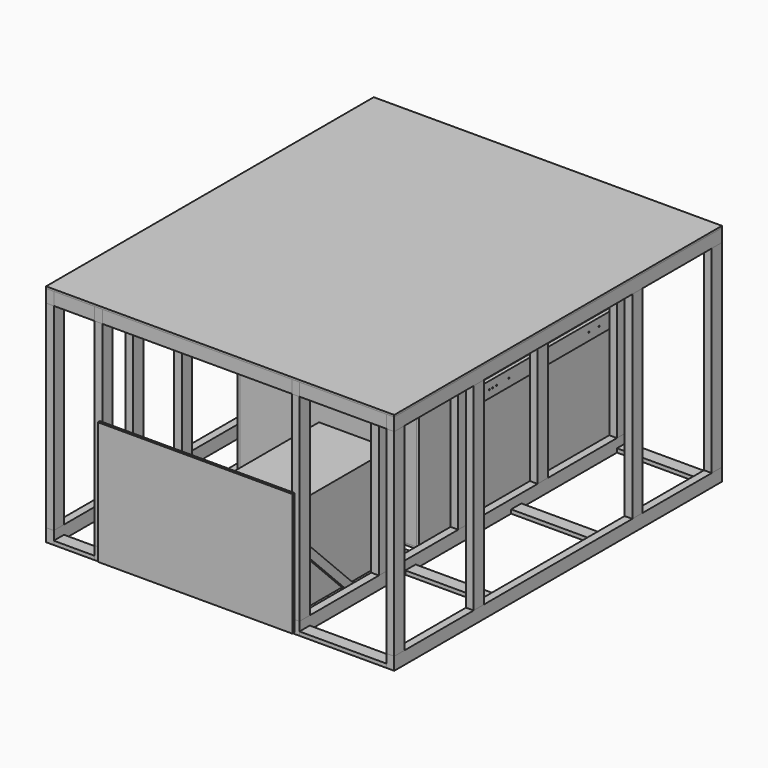
from build123d import *

# Parameters (mm, degrees)
F1_W            = 1727.2
F1_H            = 2032
F2_DEPTH        = 9.525
F3_W            = 38.1
F3_H            = 63.5
F4_DEPTH        = 2032
F5_W            = 38.1
F5_H            = 63.5
F6_DEPTH        = 981.075
F7_W            = 63.5
F7_H            = 19.05
F8_DEPTH        = 203.2
F7_W_2          = 38.1
F7_H_2          = 63.5
F7_W_3          = 19.05
F8_COPIES_COUNT = 3
F8_COPIES_PITCH = 656.166667
F9_W            = 63.5
F9_H            = 19.05
F10_DEPTH       = 431.8
F9_W_2          = 38.1
F9_H_2          = 63.5
F9_W_3          = 19.05
F11_W           = 63.5
F11_H           = 19.05
F12_DEPTH       = 939.8
F11_W_2         = 38.1
F11_H_2         = 63.5
F11_W_3         = 19.05
F13_W           = 19.05
F13_H           = 76.2
F14_DEPTH       = 914.4
F15_R           = 3.302
F16_DEPTH       = 19.05
F16_DEPTH_BACK  = 920.75
F17_W           = 901.7
F17_H           = 9.525
F18_DEPTH       = 1219.2
F19_W           = 12.7
F19_H           = 1219.2
F20_DEPTH       = 609.6
F19_W_2         = 875.792
F19_H_2         = 12.7
F21_W           = 762
F21_H           = 266.7
F22_DEPTH       = 1219.2
F24_DEPTH       = 914.4
F25_W           = 927.1
F25_H           = 9.525
F26_DEPTH       = 762
F27_W           = 965.2
F27_H           = 609.6
F28_DEPTH       = 12.7
F29_W           = 355.6
F29_H           = 635
F30_DEPTH       = 482.6
F32_DEPTH       = 19.05


# Not quite as in the source:
# - a pattern or mirror of a feature is missing from the dataset's text; its kind, count and spacing are read off the source's solid


with BuildPart() as f2:
    # F1 (on offset) → F2 (new body)
    with BuildSketch(Plane.XY.offset(1117.6)):
        Rectangle(F1_W, F1_H)
    extrude(amount=-F2_DEPTH)


with BuildPart() as f4:
    # F3 (on face) → F4 (new body, through all)
    with BuildSketch(Plane(origin=(0, 1016, 0), x_dir=(-1, 0, 0), z_dir=(0, 1, 0))):
        with Locations((-844.55, 1076.325)):
            Rectangle(F3_W, F3_H)
    extrude(amount=-F4_DEPTH)


with BuildPart() as f4b:
    # F3 (on face) → F4, piece 2 (new body, through all)
    with BuildSketch(Plane(origin=(0, 1016, 0), x_dir=(-1, 0, 0), z_dir=(0, 1, 0))):
        with Locations((844.55, 1076.325)):
            Rectangle(F3_W, F3_H)
    extrude(amount=-F4_DEPTH)


with BuildPart() as f4c:
    # F3 (on face) → F4, piece 3 (new body, through all)
    with BuildSketch(Plane(origin=(0, 1016, 0), x_dir=(-1, 0, 0), z_dir=(0, 1, 0))):
        with Locations((-844.55, 31.75)):
            Rectangle(F3_W, F3_H)
    extrude(amount=-F4_DEPTH)


with BuildPart() as f4d:
    # F3 (on face) → F4, piece 4 (new body, through all)
    with BuildSketch(Plane(origin=(0, 1016, 0), x_dir=(-1, 0, 0), z_dir=(0, 1, 0))):
        with Locations((844.55, 31.75)):
            Rectangle(F3_W, F3_H)
    extrude(amount=-F4_DEPTH)


with BuildPart() as f4e:
    # F3 (on face) → F4, piece 5 (new body, through all)
    with BuildSketch(Plane(origin=(0, 1016, 0), x_dir=(-1, 0, 0), z_dir=(0, 1, 0))):
        with Locations((-374.65, 1076.325)):
            Rectangle(F3_W, F3_H)
    extrude(amount=-F4_DEPTH)


with BuildPart() as f4f:
    # F3 (on face) → F4, piece 6 (new body, through all)
    with BuildSketch(Plane(origin=(0, 1016, 0), x_dir=(-1, 0, 0), z_dir=(0, 1, 0))):
        with Locations((603.25, 1076.325)):
            Rectangle(F3_W, F3_H)
    extrude(amount=-F4_DEPTH)


with BuildPart() as f4g:
    # F3 (on face) → F4, piece 7 (new body, through all)
    with BuildSketch(Plane(origin=(0, 1016, 0), x_dir=(-1, 0, 0), z_dir=(0, 1, 0))):
        with Locations((-374.65, 31.75)):
            Rectangle(F3_W, F3_H)
    extrude(amount=-F4_DEPTH)


with BuildPart() as f4h:
    # F3 (on face) → F4, piece 8 (new body, through all)
    with BuildSketch(Plane(origin=(0, 1016, 0), x_dir=(-1, 0, 0), z_dir=(0, 1, 0))):
        with Locations((603.25, 31.75)):
            Rectangle(F3_W, F3_H)
    extrude(amount=-F4_DEPTH)


with BuildPart() as f6:
    # F5 (on face) → F6 (new body, through all)
    with BuildSketch(Plane.XY.offset(63.5)):
        with Locations((844.55, 984.25)):
            Rectangle(F5_W, F5_H)
    extrude(amount=F6_DEPTH)


with BuildPart() as f6b:
    # F5 (on face) → F6, piece 2 (new body, through all)
    with BuildSketch(Plane.XY.offset(63.5)):
        with Locations((844.55, 492.125)):
            Rectangle(F5_W, F5_H)
    extrude(amount=F6_DEPTH)


with BuildPart() as f6c:
    # F5 (on face) → F6, piece 3 (new body, through all)
    with BuildSketch(Plane.XY.offset(63.5)):
        with Locations((844.55, -492.125)):
            Rectangle(F5_W, F5_H)
    extrude(amount=F6_DEPTH)


with BuildPart() as f6d:
    # F5 (on face) → F6, piece 4 (new body, through all)
    with BuildSketch(Plane.XY.offset(63.5)):
        with Locations((844.55, -984.25)):
            Rectangle(F5_W, F5_H)
    extrude(amount=F6_DEPTH)


with BuildPart() as f6e:
    # F5 (on face) → F6, piece 5 (new body, through all)
    with BuildSketch(Plane.XY.offset(63.5)):
        with Locations((374.65, 984.25)):
            Rectangle(F5_W, F5_H)
    extrude(amount=F6_DEPTH)


with BuildPart() as f6f:
    # F5 (on face) → F6, piece 6 (new body, through all)
    with BuildSketch(Plane.XY.offset(63.5)):
        with Locations((374.65, 492.125)):
            Rectangle(F5_W, F5_H)
    extrude(amount=F6_DEPTH)


with BuildPart() as f6g:
    # F5 (on face) → F6, piece 7 (new body, through all)
    with BuildSketch(Plane.XY.offset(63.5)):
        with Locations((374.65, 0)):
            Rectangle(F5_W, F5_H)
    extrude(amount=F6_DEPTH)


with BuildPart() as f6h:
    # F5 (on face) → F6, piece 8 (new body, through all)
    with BuildSketch(Plane.XY.offset(63.5)):
        with Locations((374.65, -492.125)):
            Rectangle(F5_W, F5_H)
    extrude(amount=F6_DEPTH)


with BuildPart() as f6i:
    # F5 (on face) → F6, piece 9 (new body, through all)
    with BuildSketch(Plane.XY.offset(63.5)):
        with Locations((374.65, -984.25)):
            Rectangle(F5_W, F5_H)
    extrude(amount=F6_DEPTH)


with BuildPart() as f6j:
    # F5 (on face) → F6, piece 10 (new body, through all)
    with BuildSketch(Plane.XY.offset(63.5)):
        with Locations((-603.25, 984.25)):
            Rectangle(F5_W, F5_H)
    extrude(amount=F6_DEPTH)


with BuildPart() as f6k:
    # F5 (on face) → F6, piece 11 (new body, through all)
    with BuildSketch(Plane.XY.offset(63.5)):
        with Locations((-603.25, 492.125)):
            Rectangle(F5_W, F5_H)
    extrude(amount=F6_DEPTH)


with BuildPart() as f6l:
    # F5 (on face) → F6, piece 12 (new body, through all)
    with BuildSketch(Plane.XY.offset(63.5)):
        with Locations((-603.25, 0)):
            Rectangle(F5_W, F5_H)
    extrude(amount=F6_DEPTH)


with BuildPart() as f6m:
    # F5 (on face) → F6, piece 13 (new body, through all)
    with BuildSketch(Plane.XY.offset(63.5)):
        with Locations((-603.25, -492.125)):
            Rectangle(F5_W, F5_H)
    extrude(amount=F6_DEPTH)


with BuildPart() as f6n:
    # F5 (on face) → F6, piece 14 (new body, through all)
    with BuildSketch(Plane.XY.offset(63.5)):
        with Locations((-603.25, -984.25)):
            Rectangle(F5_W, F5_H)
    extrude(amount=F6_DEPTH)


with BuildPart() as f6o:
    # F5 (on face) → F6, piece 15 (new body, through all)
    with BuildSketch(Plane.XY.offset(63.5)):
        with Locations((-844.55, 984.25)):
            Rectangle(F5_W, F5_H)
    extrude(amount=F6_DEPTH)


with BuildPart() as f6p:
    # F5 (on face) → F6, piece 16 (new body, through all)
    with BuildSketch(Plane.XY.offset(63.5)):
        with Locations((-844.55, 492.125)):
            Rectangle(F5_W, F5_H)
    extrude(amount=F6_DEPTH)


with BuildPart() as f6q:
    # F5 (on face) → F6, piece 17 (new body, through all)
    with BuildSketch(Plane.XY.offset(63.5)):
        with Locations((-844.55, -492.125)):
            Rectangle(F5_W, F5_H)
    extrude(amount=F6_DEPTH)


with BuildPart() as f6r:
    # F5 (on face) → F6, piece 18 (new body, through all)
    with BuildSketch(Plane.XY.offset(63.5)):
        with Locations((-844.55, -984.25)):
            Rectangle(F5_W, F5_H)
    extrude(amount=F6_DEPTH)


with BuildPart() as f8:
    # F7 (on face) → F8 (new body, through all)
    with BuildSketch(Plane(origin=(-622.3, 0, 0), x_dir=(0, -1, 0), z_dir=(-1, 0, 0))):
        with Locations((-328.0833333333, 9.525)):
            Rectangle(F7_W, F7_H)
    extrude(amount=F8_DEPTH)


with BuildPart() as f8b:
    # F7 (on face) → F8, piece 2 (new body, through all)
    with BuildSketch(Plane(origin=(-622.3, 0, 0), x_dir=(0, -1, 0), z_dir=(-1, 0, 0))):
        with Locations((-984.25, 9.525)):
            Rectangle(F7_W, F7_H)
    extrude(amount=F8_DEPTH)


with BuildPart() as f8c:
    # F7 (on face) → F8, piece 3 (new body, through all)
    with BuildSketch(Plane(origin=(-622.3, 0, 0), x_dir=(0, -1, 0), z_dir=(-1, 0, 0))):
        with Locations((996.95, 1076.325)):
            Rectangle(F7_W_2, F7_H_2)
    extrude(amount=F8_DEPTH)


with BuildPart() as f8d:
    # F7 (on face) → F8, piece 4 (new body, through all)
    with BuildSketch(Plane(origin=(-622.3, 0, 0), x_dir=(0, -1, 0), z_dir=(-1, 0, 0))):
        with Locations((661.4583333333, 1076.325)):
            Rectangle(F7_W_3, F7_H_2)
    extrude(amount=F8_DEPTH)


with BuildPart() as f8e:
    # F7 (on face) → F8, piece 5 (new body, through all)
    with BuildSketch(Plane(origin=(-622.3, 0, 0), x_dir=(0, -1, 0), z_dir=(-1, 0, 0))):
        with Locations((335.4916666667, 1076.325)):
            Rectangle(F7_W_3, F7_H_2)
    extrude(amount=F8_DEPTH)


with BuildPart() as f8f:
    # F7 (on face) → F8, piece 6 (new body, through all)
    with BuildSketch(Plane(origin=(-622.3, 0, 0), x_dir=(0, -1, 0), z_dir=(-1, 0, 0))):
        with Locations((0, 1076.325)):
            Rectangle(F7_W_2, F7_H_2)
    extrude(amount=F8_DEPTH)


with BuildPart() as f8g:
    # F7 (on face) → F8, piece 7 (new body, through all)
    with BuildSketch(Plane(origin=(-622.3, 0, 0), x_dir=(0, -1, 0), z_dir=(-1, 0, 0))):
        with Locations((-335.4916666667, 1076.325)):
            Rectangle(F7_W_3, F7_H_2)
    extrude(amount=F8_DEPTH)


with BuildPart() as f8h:
    # F7 (on face) → F8, piece 8 (new body, through all)
    with BuildSketch(Plane(origin=(-622.3, 0, 0), x_dir=(0, -1, 0), z_dir=(-1, 0, 0))):
        with Locations((-661.4583333333, 1076.325)):
            Rectangle(F7_W_3, F7_H_2)
    extrude(amount=F8_DEPTH)


with BuildPart() as f8i:
    # F7 (on face) → F8, piece 9 (new body, through all)
    with BuildSketch(Plane(origin=(-622.3, 0, 0), x_dir=(0, -1, 0), z_dir=(-1, 0, 0))):
        with Locations((-996.95, 1076.325)):
            Rectangle(F7_W_2, F7_H_2)
    extrude(amount=F8_DEPTH)


with BuildPart() as f8_copies_1:
    # F8_copies: instance of F8
    add(f8.part.moved(Location(Vector(0, -1, 0) * (1 * F8_COPIES_PITCH))))


with BuildPart() as f8_copies_2:
    # F8_copies: instance of F8
    add(f8.part.moved(Location(Vector(0, -1, 0) * (2 * F8_COPIES_PITCH))))


with BuildPart() as f10:
    # F9 (on face) → F10 (new body, through all)
    with BuildSketch(Plane.YZ.offset(393.7)):
        with Locations((-984.25, 9.525)):
            Rectangle(F9_W, F9_H)
    extrude(amount=F10_DEPTH)


with BuildPart() as f10b:
    # F9 (on face) → F10, piece 2 (new body, through all)
    with BuildSketch(Plane.YZ.offset(393.7)):
        with Locations((984.25, 9.525)):
            Rectangle(F9_W, F9_H)
    extrude(amount=F10_DEPTH)


with BuildPart() as f10c:
    # F9 (on face) → F10, piece 3 (new body, through all)
    with BuildSketch(Plane.YZ.offset(393.7)):
        with Locations((328.0833333333, 9.525)):
            Rectangle(F9_W, F9_H)
    extrude(amount=F10_DEPTH)


with BuildPart() as f10d:
    # F9 (on face) → F10, piece 4 (new body, through all)
    with BuildSketch(Plane.YZ.offset(393.7)):
        with Locations((-328.0833333333, 9.525)):
            Rectangle(F9_W, F9_H)
    extrude(amount=F10_DEPTH)


with BuildPart() as f10e:
    # F9 (on face) → F10, piece 5 (new body, through all)
    with BuildSketch(Plane.YZ.offset(393.7)):
        with Locations((996.95, 1076.325)):
            Rectangle(F9_W_2, F9_H_2)
    extrude(amount=F10_DEPTH)


with BuildPart() as f10f:
    # F9 (on face) → F10, piece 6 (new body, through all)
    with BuildSketch(Plane.YZ.offset(393.7)):
        with Locations((661.4583333333, 1076.325)):
            Rectangle(F9_W_3, F9_H_2)
    extrude(amount=F10_DEPTH)


with BuildPart() as f10g:
    # F9 (on face) → F10, piece 7 (new body, through all)
    with BuildSketch(Plane.YZ.offset(393.7)):
        with Locations((335.4916666667, 1076.325)):
            Rectangle(F9_W_3, F9_H_2)
    extrude(amount=F10_DEPTH)


with BuildPart() as f10h:
    # F9 (on face) → F10, piece 8 (new body, through all)
    with BuildSketch(Plane.YZ.offset(393.7)):
        with Locations((0, 1076.325)):
            Rectangle(F9_W_2, F9_H_2)
    extrude(amount=F10_DEPTH)


with BuildPart() as f10i:
    # F9 (on face) → F10, piece 9 (new body, through all)
    with BuildSketch(Plane.YZ.offset(393.7)):
        with Locations((-335.4916666667, 1076.325)):
            Rectangle(F9_W_3, F9_H_2)
    extrude(amount=F10_DEPTH)


with BuildPart() as f10j:
    # F9 (on face) → F10, piece 10 (new body, through all)
    with BuildSketch(Plane.YZ.offset(393.7)):
        with Locations((-661.4583333333, 1076.325)):
            Rectangle(F9_W_3, F9_H_2)
    extrude(amount=F10_DEPTH)


with BuildPart() as f10k:
    # F9 (on face) → F10, piece 11 (new body, through all)
    with BuildSketch(Plane.YZ.offset(393.7)):
        with Locations((-996.95, 1076.325)):
            Rectangle(F9_W_2, F9_H_2)
    extrude(amount=F10_DEPTH)


with BuildPart() as f12:
    # F11 (on face) → F12 (new body, through all)
    with BuildSketch(Plane(origin=(355.6, 0, 0), x_dir=(0, -1, 0), z_dir=(-1, 0, 0))):
        with Locations((-328.0833333333, 9.525)):
            Rectangle(F11_W, F11_H)
    extrude(amount=F12_DEPTH)


with BuildPart() as f12b:
    # F11 (on face) → F12, piece 2 (new body, through all)
    with BuildSketch(Plane(origin=(355.6, 0, 0), x_dir=(0, -1, 0), z_dir=(-1, 0, 0))):
        with Locations((-984.25, 9.525)):
            Rectangle(F11_W, F11_H)
    extrude(amount=F12_DEPTH)


with BuildPart() as f12c:
    # F11 (on face) → F12, piece 3 (new body, through all)
    with BuildSketch(Plane(origin=(355.6, 0, 0), x_dir=(0, -1, 0), z_dir=(-1, 0, 0))):
        with Locations((996.95, 1076.325)):
            Rectangle(F11_W_2, F11_H_2)
    extrude(amount=F12_DEPTH)


with BuildPart() as f12d:
    # F11 (on face) → F12, piece 4 (new body, through all)
    with BuildSketch(Plane(origin=(355.6, 0, 0), x_dir=(0, -1, 0), z_dir=(-1, 0, 0))):
        with Locations((-996.95, 1076.325)):
            Rectangle(F11_W_2, F11_H_2)
    extrude(amount=F12_DEPTH)


with BuildPart() as f12e:
    # F11 (on face) → F12, piece 5 (new body, through all)
    with BuildSketch(Plane(origin=(355.6, 0, 0), x_dir=(0, -1, 0), z_dir=(-1, 0, 0))):
        with Locations((-661.4583333333, 1076.325)):
            Rectangle(F11_W_3, F11_H_2)
    extrude(amount=F12_DEPTH)


with BuildPart() as f12f:
    # F11 (on face) → F12, piece 6 (new body, through all)
    with BuildSketch(Plane(origin=(355.6, 0, 0), x_dir=(0, -1, 0), z_dir=(-1, 0, 0))):
        with Locations((-335.4916666667, 1076.325)):
            Rectangle(F11_W_3, F11_H_2)
    extrude(amount=F12_DEPTH)


with BuildPart() as f12g:
    # F11 (on face) → F12, piece 7 (new body, through all)
    with BuildSketch(Plane(origin=(355.6, 0, 0), x_dir=(0, -1, 0), z_dir=(-1, 0, 0))):
        with Locations((0, 1076.325)):
            Rectangle(F11_W_2, F11_H_2)
    extrude(amount=F12_DEPTH)


with BuildPart() as f12h:
    # F11 (on face) → F12, piece 8 (new body, through all)
    with BuildSketch(Plane(origin=(355.6, 0, 0), x_dir=(0, -1, 0), z_dir=(-1, 0, 0))):
        with Locations((335.4916666667, 1076.325)):
            Rectangle(F11_W_3, F11_H_2)
    extrude(amount=F12_DEPTH)


with BuildPart() as f12i:
    # F11 (on face) → F12, piece 9 (new body, through all)
    with BuildSketch(Plane(origin=(355.6, 0, 0), x_dir=(0, -1, 0), z_dir=(-1, 0, 0))):
        with Locations((661.4583333333, 1076.325)):
            Rectangle(F11_W_3, F11_H_2)
    extrude(amount=F12_DEPTH)


with BuildPart() as f14:
    # F13 (on face) → F14 (new body)
    with BuildSketch(Plane(origin=(0, 1016, 0), x_dir=(-1, 0, 0), z_dir=(0, 1, 0))):
        with Locations((-346.075, 565.15)):
            Rectangle(F13_W, F13_H)
    extrude(amount=-F14_DEPTH)


with BuildPart() as f14b:
    # F13 (on face) → F14, piece 2 (new body)
    with BuildSketch(Plane(origin=(0, 1016, 0), x_dir=(-1, 0, 0), z_dir=(0, 1, 0))):
        with Locations((574.675, 565.15)):
            Rectangle(F13_W, F13_H)
    extrude(amount=-F14_DEPTH)


with BuildPart() as f16_tool:
    # F15 (on face) → F16 (new body, two sides)
    with BuildSketch(Plane(origin=(336.55, 0, 0), x_dir=(0, -1, 0), z_dir=(-1, 0, 0))) as f16_sk:
        with Locations((-977.9, 565.15)):
            Circle(F15_R)
        with Locations((-889, 565.15)):
            Circle(F15_R)
        with Locations((-825.5, 565.15)):
            Circle(F15_R)
        with Locations((-495.3, 565.15)):
            Circle(F15_R)
        with Locations((-330.2, 565.15)):
            Circle(F15_R)
        with Locations((-254, 565.15)):
            Circle(F15_R)
        with Locations((-228.6, 565.15)):
            Circle(F15_R)
        with Locations((-208.28, 565.15)):
            Circle(F15_R)
    extrude(amount=-F16_DEPTH)
    extrude(f16_sk.sketch, amount=F16_DEPTH_BACK)


with BuildPart() as f14_1:
    add(f14.part)

    # F16: cut by f16_tool
    add(f16_tool.part, mode=Mode.SUBTRACT)


with BuildPart() as f14b_1:
    add(f14b.part)

    # F16: cut by f16_tool
    add(f16_tool.part, mode=Mode.SUBTRACT)


with BuildPart() as f18:
    # F17 (on face) → F18 (new body)
    with BuildSketch(Plane(origin=(0, 1016, 0), x_dir=(-1, 0, 0), z_dir=(0, 1, 0))):
        with Locations((114.3, 30.1625)):
            Rectangle(F17_W, F17_H)
    extrude(amount=-F18_DEPTH)


with BuildPart() as f20:
    # F19 (on face) → F20 (new body)
    with BuildSketch(Plane.XY.offset(34.925)):
        with Locations((330.2, 406.4)):
            Rectangle(F19_W, F19_H)
    extrude(amount=F20_DEPTH)


with BuildPart() as f20b:
    # F19 (on face) → F20, piece 2 (new body)
    with BuildSketch(Plane.XY.offset(34.925)):
        with Locations((-114.3, -196.85)):
            Rectangle(F19_W_2, F19_H_2)
    extrude(amount=F20_DEPTH)


with BuildPart() as f20c:
    # F19 (on face) → F20, piece 3 (new body)
    with BuildSketch(Plane.XY.offset(34.925)):
        with Locations((-558.8, 406.4)):
            Rectangle(F19_W, F19_H)
    extrude(amount=F20_DEPTH)


with BuildPart() as f20d:
    # F19 (on face) → F20, piece 4 (new body)
    with BuildSketch(Plane.XY.offset(34.925)):
        with Locations((-114.3, 1009.65)):
            Rectangle(F19_W_2, F19_H_2)
    extrude(amount=F20_DEPTH)


with BuildPart() as f22:
    # F21 (on face) → F22 (new body)
    with BuildSketch(Plane(origin=(0, 1016, 0), x_dir=(-1, 0, 0), z_dir=(0, 1, 0))):
        with Locations((114.3000000002, 898.525)):
            Rectangle(F21_W, F21_H)
    extrude(amount=-F22_DEPTH)


with BuildPart() as f24:
    # F23 (on face) → F24 (new body)
    with BuildSketch(Plane(origin=(0, 1016, 0), x_dir=(-1, 0, 0), z_dir=(0, 1, 0))):
        Polygon((-279.4, 758.825), (-279.4, 765.175), (-355.6, 765.175), (-355.6, 688.975), (-349.25, 688.975), (-349.25, 758.825), align=None)
    extrude(amount=-F24_DEPTH)


with BuildPart() as f24b:
    # F23 (on face) → F24, piece 2 (new body)
    with BuildSketch(Plane(origin=(0, 1016, 0), x_dir=(-1, 0, 0), z_dir=(0, 1, 0))):
        Polygon((577.85, 758.825), (577.85, 688.975), (584.2, 688.975), (584.2, 765.175), (508, 765.175), (508, 758.825), align=None)
    extrude(amount=-F24_DEPTH)


with BuildPart() as f26:
    # F25 (on face) → F26 (new body)
    with BuildSketch(Plane.XZ.offset(1016)):
        with Locations((-114.3, 36.5125)):
            Rectangle(F25_W, F25_H)
    extrude(amount=-F26_DEPTH)


with BuildPart() as f28:
    # F27 (on face) → F28 (new body)
    with BuildSketch(Plane.XZ.offset(1016)):
        with Locations((-114.3, 311.15)):
            Rectangle(F27_W, F27_H)
    extrude(amount=F28_DEPTH)


with BuildPart() as f30:
    # F29 (on face) → F30 (new body)
    with BuildSketch(Plane.XY.offset(41.275)):
        with Locations((139.7, -673.1)):
            Rectangle(F29_W, F29_H)
    extrude(amount=F30_DEPTH)


with BuildPart() as f32:
    # F31 (on face) → F32 (new body)
    with BuildSketch(Plane.YZ.offset(349.25)):
        Polygon((-663.4815367264, 41.275), (-609.6, 41.275), (-1016, 447.675), (-1016, 393.7934632736), align=None)
    extrude(amount=-F32_DEPTH)


with BuildPart() as f35_1:
    # F35: instance of F32
    add(f32.part.mirror(Plane(origin=(-114.3, -673.1, 282.575), x_dir=(0, -1, 0), z_dir=(-1, 0, 0))))


solid = Compound([f2.part, f4.part, f4b.part, f4c.part, f4d.part, f4e.part, f4f.part, f4g.part, f4h.part, f6.part, f6b.part, f6c.part, f6d.part, f6e.part, f6f.part, f6g.part, f6h.part, f6i.part, f6j.part, f6k.part, f6l.part, f6m.part, f6n.part, f6o.part, f6p.part, f6q.part, f6r.part, f8.part, f8b.part, f8c.part, f8d.part, f8e.part, f8f.part, f8g.part, f8h.part, f8i.part, f8_copies_1.part, f8_copies_2.part, f10.part, f10b.part, f10c.part, f10d.part, f10e.part, f10f.part, f10g.part, f10h.part, f10i.part, f10j.part, f10k.part, f12.part, f12b.part, f12c.part, f12d.part, f12e.part, f12f.part, f12g.part, f12h.part, f12i.part, f14_1.part, f14b_1.part, f18.part, f20.part, f20b.part, f20c.part, f20d.part, f22.part, f24.part, f24b.part, f26.part, f28.part, f30.part, f32.part, f35_1.part])
